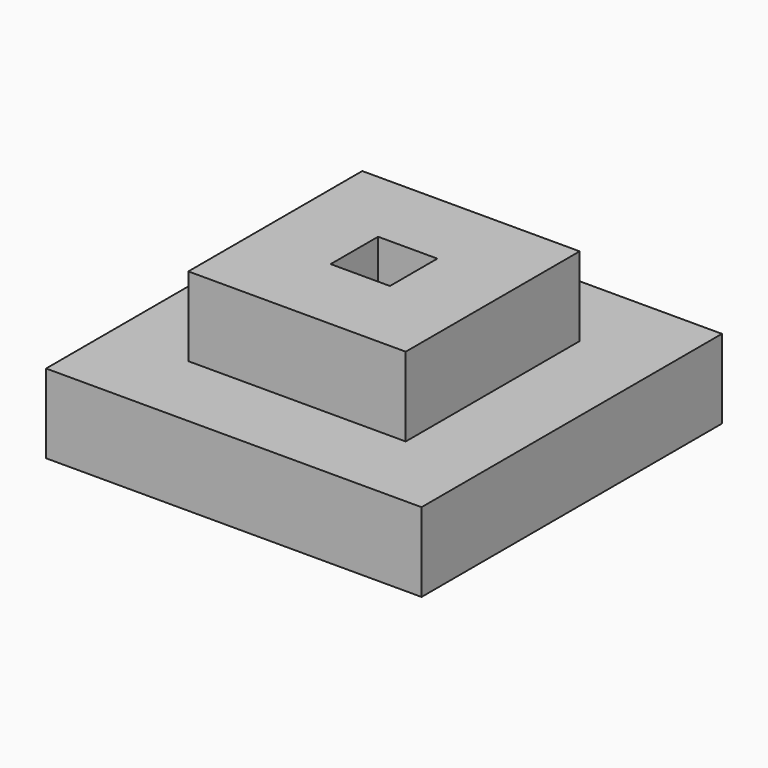
from build123d import *

# Parameters (mm, degrees)
F0_W     = 45.24375
F0_H     = 45.24375
F0_W_2   = 26.19375
F0_H_2   = 26.19375
F1_DEPTH = 9.525
F0_W_3   = 7.14375
F0_H_3   = 7.14375
F2_DEPTH = 19.05
F3_DEPTH = 6.35


# Not quite as in the source:
# - a length typed as a fraction of an inch, garbled in the dataset ("3 / 203.2 mm" for 3/8 in), is restored


with BuildPart() as f1:
    # F0 (on Top) → F1 (new body)
    with BuildSketch(Plane.XY):
        Rectangle(F0_W, F0_H)
        Rectangle(F0_W_2, F0_H_2, mode=Mode.SUBTRACT)
    extrude(amount=F1_DEPTH)

    # F0 (on Top) → F2 (join)
    with BuildSketch(Plane.XY):
        Rectangle(F0_W_2, F0_H_2)
        Rectangle(F0_W_3, F0_H_3, mode=Mode.SUBTRACT)
    extrude(amount=F2_DEPTH)

    # F0 (on Top) → F3 (join)
    with BuildSketch(Plane.XY):
        Rectangle(F0_W_3, F0_H_3)
    extrude(amount=F3_DEPTH)


solid = f1.part
